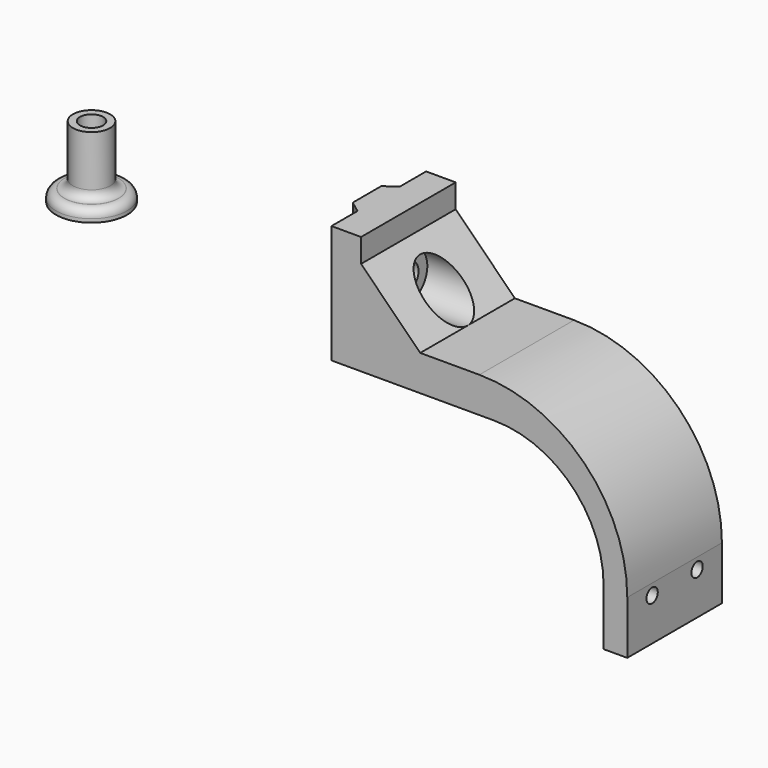
from build123d import *

# Parameters (mm, degrees)
F0_W       = 4
F0_H       = 28
F1_DEPTH   = 20
F2_R       = 2.15
F3_DEPTH   = 50.001
F4_START   = -5
F2_R_2     = 4
F4_DEPTH   = 45.001
F6_D       = 2.4
F6_DEPTH   = 8
F6_TIP     = 0.7210327428
F2_W       = 9
F2_H       = 4
F7_DEPTH   = 2
F8_SIZE2   = 1.49999
F8_SIZE    = 1.99999
F8_2_SIZE2 = 1.49999
F8_2_SIZE  = 1.99999
F9_SIZE2   = 1.49999
F9_SIZE    = 1.99999
F9_2_SIZE2 = 1.49999
F9_2_SIZE  = 1.99999
F11_DEPTH  = 2
F12_R      = 18.5
F13_R      = 25
F14_R      = 6
F15_DEPTH  = 2
F16_R      = 3.15
F16_R_2    = 1.95
F17_DEPTH  = 10
F18_R      = 1.4


# Not quite as in the source:
# - a fillet or chamfer is up to 0.001 mm smaller than in the source, because OpenCascade refuses the exact size
# - a feature names something its author has since deleted; it is built from what else it names


with BuildPart() as f1:
    # F0 (on Front) → F1 (new body)
    with BuildSketch(Plane.XZ):
        Polygon((0, 20), (0, 0), (46, 0), (50, 0), (50, 6), (15, 6), (5, 16), (5, 20), align=None)
        with Locations((48, -14)):
            Rectangle(F0_W, F0_H)
    extrude(amount=F1_DEPTH)

    # F2 (on face) → F3 (cut, through all)
    with BuildSketch(Plane(origin=(0, 0, 0), x_dir=(0, -1, 0), z_dir=(-1, 0, 0))):
        with Locations((10, 10)):
            Circle(F2_R)
    extrude(amount=-F3_DEPTH, mode=Mode.SUBTRACT)

    # F2 (on face) → F4 (cut)
    with BuildSketch(Plane(origin=(0, 0, 0), x_dir=(0, -1, 0), z_dir=(-1, 0, 0)).offset(F4_START)):
        with Locations((10, 10)):
            Circle(F2_R_2)
        with Locations((10, 10)):
            Circle(F2_R, mode=Mode.SUBTRACT)
    extrude(amount=-F4_DEPTH, mode=Mode.SUBTRACT)

    # F6
    with Locations(Plane.YZ.offset(50)):
        with Locations((-14.75, -20.85), (-5.25, -20.85)):
            Hole(F6_D / 2, depth=F6_DEPTH)
            with Locations((0, 0, -(F6_DEPTH + F6_TIP / 2))):  # 118° drill point
                Cone(0, F6_D / 2, F6_TIP, mode=Mode.SUBTRACT)

    # F2 (on face) → F7 (join)
    with BuildSketch(Plane(origin=(0, 0, 0), x_dir=(0, -1, 0), z_dir=(-1, 0, 0))):
        with Locations((10, 2)):
            Rectangle(F2_W, F2_H)
        with Locations((10, 18)):
            Rectangle(F2_W, F2_H)
    extrude(amount=F7_DEPTH)

    # F8 (size 2 and 1.5 in the source; OpenCascade refuses exactly that, so slightly less here)
    f8_edges = [f1.edges().sort_by_distance(p)[0] for p in [
        (-2, -5.5, 2),
    ]]
    f8_side = f1.faces().sort_by_distance((-1, -5.5, 2))[0]
    chamfer(f8_edges, length=F8_SIZE, length2=F8_SIZE2, reference=f8_side)

    # F8#2 (size 2 and 1.5 in the source; OpenCascade refuses exactly that, so slightly less here)
    f8_2_edges = [f1.edges().sort_by_distance(p)[0] for p in [
        (-2, -14.5, 2),
    ]]
    f8_2_side = f1.faces().sort_by_distance((-1, -14.5, 2))[0]
    chamfer(f8_2_edges, length=F8_2_SIZE, length2=F8_2_SIZE2, reference=f8_2_side)

    # F9 (size 2 and 1.5 in the source; OpenCascade refuses exactly that, so slightly less here)
    f9_edges = [f1.edges().sort_by_distance(p)[0] for p in [
        (-2, -14.5, 18),
    ]]
    f9_side = f1.faces().sort_by_distance((-1, -14.5, 18))[0]
    chamfer(f9_edges, length=F9_SIZE, length2=F9_SIZE2, reference=f9_side)

    # F9#2 (size 2 and 1.5 in the source; OpenCascade refuses exactly that, so slightly less here)
    f9_2_edges = [f1.edges().sort_by_distance(p)[0] for p in [
        (-2, -5.5, 18),
    ]]
    f9_2_side = f1.faces().sort_by_distance((-1, -5.5, 18))[0]
    chamfer(f9_2_edges, length=F9_2_SIZE, length2=F9_2_SIZE2, reference=f9_2_side)

    # F10 (on face) → F11 (cut)
    with BuildSketch(Plane(origin=(46, 0, 0), x_dir=(0, -1, 0), z_dir=(-1, 0, 0))):
        Polygon((6.5490381057, -23.1), (7.8480762114, -20.85), (6.5490381057, -18.6), (3.9509618943, -18.6), (2.6519237886, -20.85), (3.9509618943, -23.1), align=None)
        Polygon((12.1519237886, -20.85), (13.4509618943, -23.1), (16.0490381057, -23.1), (17.3480762114, -20.85), (16.0490381057, -18.6), (13.4509618943, -18.6), align=None)
    extrude(amount=-F11_DEPTH, mode=Mode.SUBTRACT)

    # F12
    f12_edges = [f1.edges().sort_by_distance(p)[0] for p in [
        (46, -10, 0),
    ]]
    fillet(f12_edges, radius=F12_R)

    # F13
    f13_edges = [f1.edges().sort_by_distance(p)[0] for p in [
        (50, -10, 6),
    ]]
    fillet(f13_edges, radius=F13_R)


with BuildPart() as f15:
    # F14 (on Top) → F15 (new body)
    with BuildSketch(Plane.XY):
        with Locations((-53.0685186386, -4.3631289154)):
            Circle(F14_R)
    extrude(amount=F15_DEPTH)

    # F16 (on face) → F17 (join)
    with BuildSketch(Plane.XY.offset(2)):
        with Locations((-53.0685186386, -4.3631289154)):
            Circle(F16_R)
        with Locations((-53.0685186386, -4.3631289154)):
            Circle(F16_R_2, mode=Mode.SUBTRACT)
    extrude(amount=F17_DEPTH)

    # F18
    f18_edges = [f15.edges().sort_by_distance(p)[0] for p in [
        (-56.218519, -4.363129, 2),
        (-59.068519, -4.363129, 2),
    ]]
    fillet(f18_edges, radius=F18_R)


solid = Compound([f1.part, f15.part])
